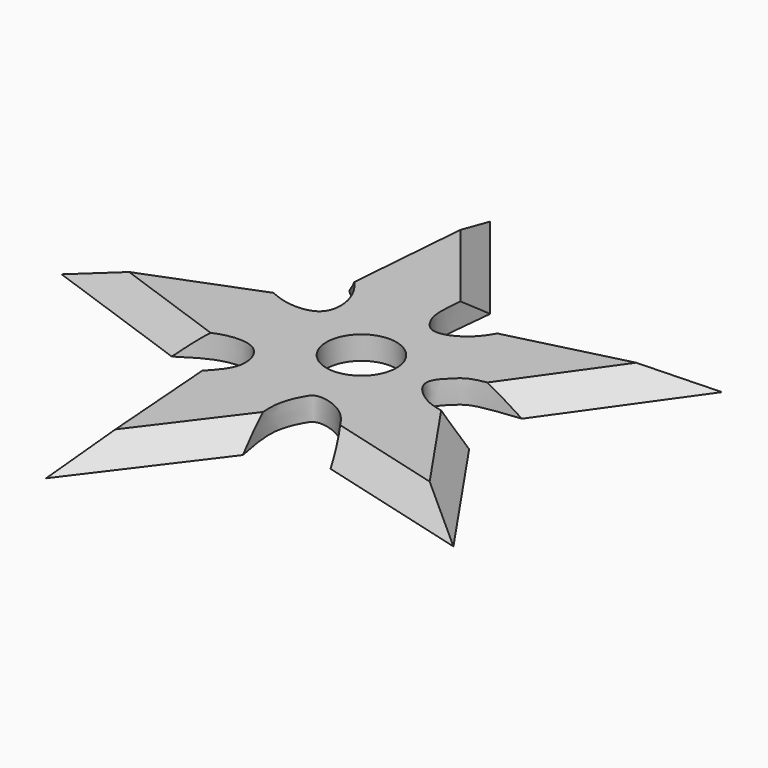
from build123d import *

# Parameters (mm, degrees)
F1_DEPTH = 2
F2_SIZE  = 1.99999
F4_D     = 6


# Not quite as in the source:
# - a fillet or chamfer is up to 0.001 mm smaller than in the source, because OpenCascade refuses the exact size


with BuildPart() as f1:
    # F0 (on Top) → F1 (new body)
    with BuildSketch(Plane.XY):
        with BuildLine():
            Line((-6.070732047, 22.9513901076), (-7.1661561031, 9.2087939751))
            add(Edge.make_bspline(
                [(-10.8183338371, 4.072241369), (-9.5749830205, 3.3108681768), (-7.3147246833, 1.9267856777), (-3.6193330593, 2.323879706), (-3.8736126343, 6.3110586072), (-5.9992796786, 8.181837424), (-7.1661561031, 9.2087939751)],
                knots=[0, 0, 0, 0, 0.2710094176, 0.4926616748, 0.721498655, 1, 1, 1, 1], degree=3))
            Line((-10.8183338371, 4.072241369), (-23.7063266087, -0.9532651191))
            Line((-23.7063266087, -0.9532651191), (-10.4941075873, -5.6545452478))
            add(Edge.make_bspline(
                [(-10.4941075873, -5.6545452478), (-9.4938612527, -5.0046237284), (-7.5990391104, -3.7734413255), (-4.2858275376, -3.7917280391), (-3.3433653275, -6.5786033893), (-4.5476101592, -8.3403208195), (-5.9073550155, -9.6570884675), (-6.7070025438, -10.4037433444), (-7.0897310874, -10.7611084628)],
                knots=[0, 0, 0, 0, 0.2047671487, 0.3879017737, 0.5554252257, 0.7107538026, 0.8615605352, 1, 1, 1, 1], degree=3))
            Line((-7.0897310874, -10.7611084628), (-6.0359964333, -24.702837204))
            Line((-6.0359964333, -24.702837204), (2.1507161547, -13.8412582744))
            add(Edge.make_bspline(
                [(2.1507161547, -13.8412582744), (1.857437852, -12.3709258177), (1.3508773092, -9.8313161697), (2.3957995803, -7.6684734808), (3.0110019697, -6.7670125475), (5.8159743775, -7.4801379246), (7.4501009355, -10.1557150048), (7.8283613318, -11.2679488073), (7.9867886511, -11.7337872122)],
                knots=[0, 0, 0, 0, 0.2247705341, 0.3882315284, 0.4906474402, 0.664362762, 0.8594245965, 1, 1, 1, 1], degree=3))
            Line((7.9867886511, -11.7337872122), (21.4421775791, -15.3813331802))
            Line((21.4421775791, -15.3813331802), (13.4529346897, -3.7091881875))
            add(Edge.make_bspline(
                [(13.4529346897, 1.9505254996), (11.9323407983, 1.79071702), (9.5330178877, 1.5385575522), (8.581661333, 0.6216498394), (6.8511425341, -1.0519539126), (9.4923390362, -3.4928584716), (12.2268542531, -3.6020610918), (13.107191535, -3.6789793538), (13.4529346897, -3.7091881875)],
                knots=[0, 0, 0, 0, 0.2219857691, 0.3502681055, 0.5009951592, 0.691693444, 0.8789158616, 1, 1, 1, 1], degree=3))
            Line((13.4529346897, 1.9505254996), (21.5007144708, 13.33170683))
            Line((21.5007144708, 13.33170683), (8.0718742184, 9.9506860604))
            add(Edge.make_bspline(
                [(2.294327212, 12.4950657049), (2.1198852992, 10.9346638034), (1.8320041162, 8.3595352793), (1.8961121506, 6.5524820747), (3.1599495173, 4.614552865), (6.0828787964, 6.0160070097), (7.1855048229, 8.2606927811), (7.7920128495, 9.4170893061), (8.0718742184, 9.9506860604)],
                knots=[0, 0, 0, 0, 0.2205766948, 0.364017333, 0.5063227579, 0.6820195585, 0.8532740908, 1, 1, 1, 1], degree=3))
            Line((2.294327212, 12.4950657049), (-6.070732047, 22.9513901076))
        make_face()
    extrude(amount=F1_DEPTH)

    # F2 (size 2 in the source; OpenCascade refuses exactly that, so slightly less here)
    f2_edges = [f1.edges().sort_by_distance(p)[0] for p in [
        (-1.888202, 17.723228, 2),
        (-6.618444, 16.080092, 2),
        (17.476825, 7.641116, 2),
        (14.786294, 11.641196, 2),
        (17.447556, -9.545261, 2),
        (14.714483, -13.55756, 2),
        (-1.94264, -19.272048, 2),
        (-6.562864, -17.731973, 2),
        (-17.100217, -3.303905, 2),
        (-17.26233, 1.559488, 2),
    ]]
    chamfer(f2_edges, length=F2_SIZE)

    # F4 (through all)
    with Locations(Plane(origin=(0, 0, 0), x_dir=(1, 0, 0), z_dir=(0, 0, -1))):
        with Locations((1.6917608845, 0.5521112873)):
            Hole(F4_D / 2)


solid = f1.part
